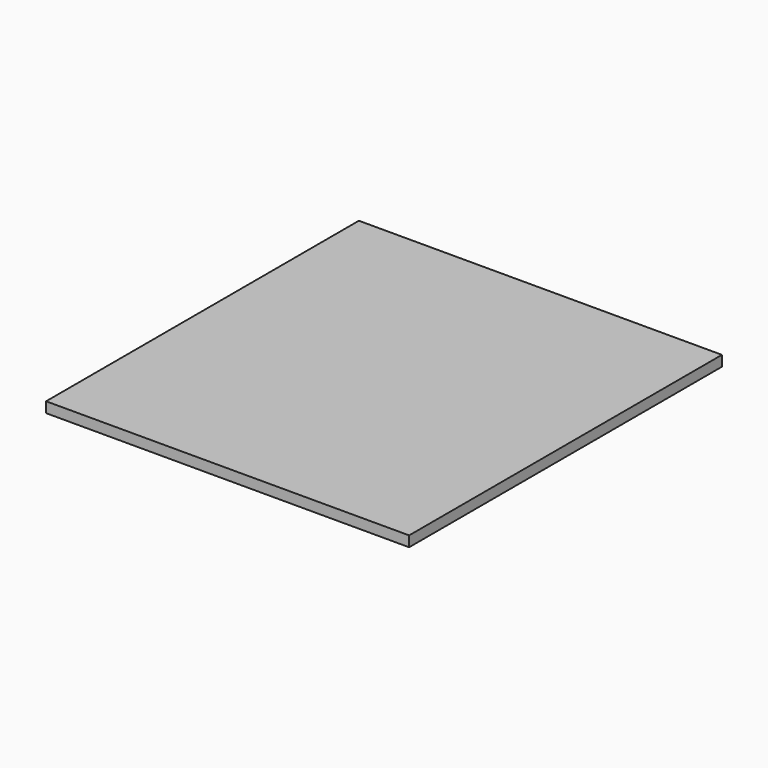
from build123d import *

# Parameters (mm, degrees)
F1_W     = 660.4
F1_H     = 711.2
F2_DEPTH = 19.05


# Not quite as in the source:
# - a variable given as a bare number and used for a length is read in inches; the dataset says mm whatever the document's units were


with BuildPart() as f2:
    # F1 (on Top) → F2 (new body)
    with BuildSketch(Plane.XY):
        Rectangle(F1_W, F1_H)
    extrude(amount=F2_DEPTH)


solid = f2.part
